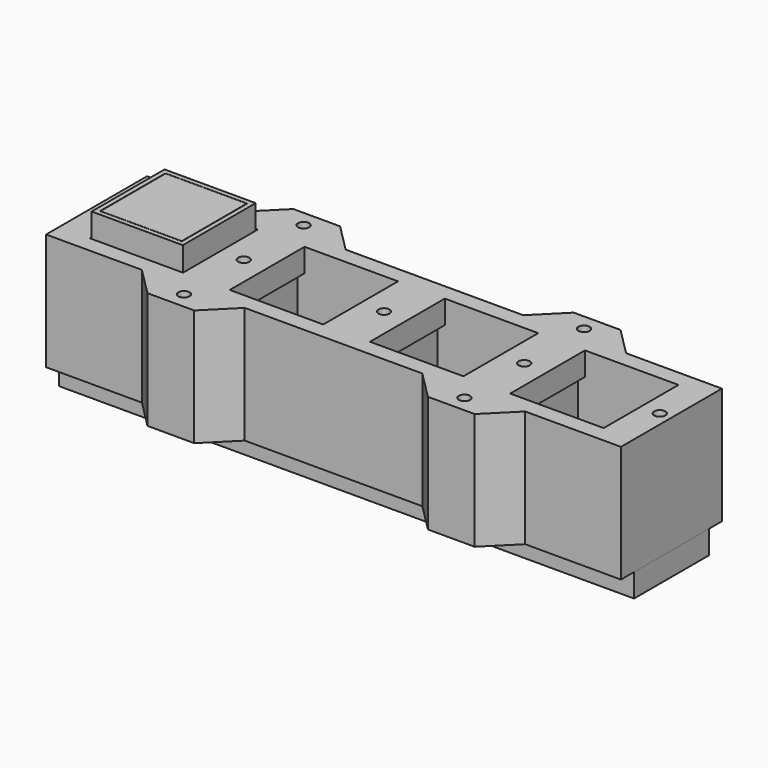
from build123d import *

# Parameters (mm, degrees)
F0_W      = 19.5
F0_H      = 19.5
F1_DEPTH  = 13
F2_W      = 19.5
F2_H      = 19.5
F2_W_2    = 17.5
F2_H_2    = 17.5
F3_DEPTH  = 6
F5_DEPTH  = 4
F6_R      = 3.1
F7_DEPTH  = 19
F8_W      = 1.5
F8_H      = 19.5
F9_DEPTH  = 9
F10_R     = 2.55
F11_DEPTH = 3
F13_W     = 10
F13_H     = 6
F13_W_2   = 20
F13_H_2   = 20
F14_DEPTH = 25
F15_W     = 23
F15_H     = 20
F16_DEPTH = 20
F17_R     = 1.2
F18_DEPTH = 30
F19_R     = 1.2
F20_DEPTH = 30.001
F21_W     = 123
F21_H     = 20
F21_R     = 2.75
F21_R_2   = 1.5
F21_R_3   = 4
F22_DEPTH = 5
F23_SIZE  = 5.99999
F25_W     = 3
F25_H     = 8
F25_H_2   = 3
F25_W_2   = 9.5
F26_DEPTH = 11
F27_W     = 17.4
F27_H     = 17.4
F28_DEPTH = 2


# Not quite as in the source:
# - a fillet or chamfer is up to 0.001 mm smaller than in the source, because OpenCascade refuses the exact size


with BuildPart() as f1:
    # F0 (on Top) → F1 (new body)
    with BuildSketch(Plane.XY):
        Rectangle(F0_W, F0_H)
    extrude(amount=F1_DEPTH)

    # F2 (on face) → F3 (join)
    with BuildSketch(Plane.XY.offset(13)):
        Rectangle(F2_W, F2_H)
        Rectangle(F2_W_2, F2_H_2, mode=Mode.SUBTRACT)
    extrude(amount=F3_DEPTH)

    # F4 (on face) → F5 (join)
    with BuildSketch(Plane.XY.offset(13)):
        Polygon((0.5, 8.75), (-0.5, 8.75), (-0.5, 0.5), (-8.75, 0.5), (-8.75, -0.5), (-0.5, -0.5), (-0.5, -8.75), (0.5, -8.75), (0.5, -0.5), (8.75, -0.5), (8.75, 0.5), (0.5, 0.5), align=None)
    extrude(amount=F5_DEPTH)

    # F6 (on face) → F7 (cut)
    with BuildSketch(Plane.XY.offset(13)):
        with Locations((-4.5, 4.5)):
            Circle(F6_R)
        with Locations((-4.5, -4.5)):
            Circle(F6_R)
        with Locations((4.5, 4.5)):
            Circle(F6_R)
        with Locations((4.5, -4.5)):
            Circle(F6_R)
    extrude(amount=-F7_DEPTH, mode=Mode.SUBTRACT)

    # F8 (on face) → F9 (join)
    with BuildSketch(Plane(origin=(0, 0, 0), x_dir=(1, 0, 0), z_dir=(0, 0, -1))):
        with Locations((-10.5, 0)):
            Rectangle(F8_W, F8_H)
        with Locations((10.5, 0)):
            Rectangle(F8_W, F8_H)
    extrude(amount=-F9_DEPTH)

    # F10 (on face) → F11 (cut)
    with BuildSketch(Plane(origin=(0, 0, 0), x_dir=(1, 0, 0), z_dir=(0, 0, -1))):
        Circle(F10_R)
    extrude(amount=-F11_DEPTH, mode=Mode.SUBTRACT)


with BuildPart() as f14:
    # F13 (on offset) → F14 (new body)
    with BuildSketch(Plane.XY.offset(14)):
        with Locations((15, 16.5)):
            Rectangle(F13_W, F13_H)
        Polygon((20, 13.5), (10, 13.5), (-16.5, 13.5), (-16.5, -13.5), (10, -13.5), (20, -13.5), (70, -13.5), (80, -13.5), (106.5, -13.5), (106.5, 13.5), (80, 13.5), (70, 13.5), align=None)
        Rectangle(F13_W_2, F13_H_2, mode=Mode.SUBTRACT)
        with Locations((30, 0)):
            Rectangle(F13_W_2, F13_H_2, mode=Mode.SUBTRACT)
        with Locations((60, 0)):
            Rectangle(F13_W_2, F13_H_2, mode=Mode.SUBTRACT)
        with Locations((90, 0)):
            Rectangle(F13_W_2, F13_H_2, mode=Mode.SUBTRACT)
        with Locations((75, 16.5)):
            Rectangle(F13_W, F13_H)
        with Locations((15, -16.5)):
            Rectangle(F13_W, F13_H)
        with Locations((75, -16.5)):
            Rectangle(F13_W, F13_H)
    extrude(amount=-F14_DEPTH)

    # F15 (on face) → F16 (cut)
    with BuildSketch(Plane(origin=(0, 0, -11), x_dir=(1, 0, 0), z_dir=(0, 0, -1))):
        Rectangle(F15_W, F15_H)
        with Locations((30, 0)):
            Rectangle(F15_W, F15_H)
        with Locations((60, 0)):
            Rectangle(F15_W, F15_H)
        with Locations((90, 0)):
            Rectangle(F15_W, F15_H)
    extrude(amount=-F16_DEPTH, mode=Mode.SUBTRACT)

    # F17 (on face) → F18 (cut)
    with BuildSketch(Plane.XY.offset(14)):
        with Locations((15, 16)):
            Circle(F17_R)
        with Locations((15, -16)):
            Circle(F17_R)
        with Locations((75, 16)):
            Circle(F17_R)
        with Locations((75, -16)):
            Circle(F17_R)
    extrude(amount=-F18_DEPTH, mode=Mode.SUBTRACT)

    # F19 (on face) → F20 (cut, through all)
    with BuildSketch(Plane(origin=(0, 0, -11), x_dir=(1, 0, 0), z_dir=(0, 0, -1))):
        with Locations((-14, 0)):
            Circle(F19_R)
        with Locations((15, 0)):
            Circle(F19_R)
        with Locations((45, 0)):
            Circle(F19_R)
        with Locations((75, 0)):
            Circle(F19_R)
        with Locations((104, 0)):
            Circle(F19_R)
    extrude(amount=-F20_DEPTH, mode=Mode.SUBTRACT)

    # F23 (size 6 in the source; OpenCascade refuses exactly that, so slightly less here)
    f23_edges = [f14.edges().sort_by_distance(p)[0] for p in [
        (10, -13.5, 1.5),
        (20, -13.5, 1.5),
        (70, -13.5, 1.5),
        (80, -13.5, 1.5),
        (10, 13.5, 1.5),
        (20, 13.5, 1.5),
        (70, 13.5, 1.5),
        (80, 13.5, 1.5),
    ]]
    chamfer(f23_edges, length=F23_SIZE)


with BuildPart() as f22:
    # F21 (on face) → F22 (new body)
    with BuildSketch(Plane(origin=(0, 0, -11), x_dir=(1, 0, 0), z_dir=(0, 0, -1))):
        with Locations((45, 0)):
            Rectangle(F21_W, F21_H)
        with Locations((-5.5, -5.5)):
            Circle(F21_R, mode=Mode.SUBTRACT)
        with Locations((5.5, -5.5)):
            Circle(F21_R, mode=Mode.SUBTRACT)
        with Locations((24.5, -5.5)):
            Circle(F21_R, mode=Mode.SUBTRACT)
        with Locations((35.5, -5.5)):
            Circle(F21_R, mode=Mode.SUBTRACT)
        with Locations((54.5, -5.5)):
            Circle(F21_R, mode=Mode.SUBTRACT)
        with Locations((65.5, -5.5)):
            Circle(F21_R, mode=Mode.SUBTRACT)
        with Locations((84.5, -5.5)):
            Circle(F21_R, mode=Mode.SUBTRACT)
        with Locations((95.5, -5.5)):
            Circle(F21_R, mode=Mode.SUBTRACT)
        with Locations((-14, 0)):
            Circle(F21_R_2, mode=Mode.SUBTRACT)
        Circle(F21_R_3, mode=Mode.SUBTRACT)
        with Locations((15, 0)):
            Circle(F21_R_2, mode=Mode.SUBTRACT)
        with Locations((30, 0)):
            Circle(F21_R_3, mode=Mode.SUBTRACT)
        with Locations((-5.5, 5.5)):
            Circle(F21_R, mode=Mode.SUBTRACT)
        with Locations((5.5, 5.5)):
            Circle(F21_R, mode=Mode.SUBTRACT)
        with Locations((24.5, 5.5)):
            Circle(F21_R, mode=Mode.SUBTRACT)
        with Locations((35.5, 5.5)):
            Circle(F21_R, mode=Mode.SUBTRACT)
        with Locations((45, 0)):
            Circle(F21_R_2, mode=Mode.SUBTRACT)
        with Locations((60, 0)):
            Circle(F21_R_3, mode=Mode.SUBTRACT)
        with Locations((75, 0)):
            Circle(F21_R_2, mode=Mode.SUBTRACT)
        with Locations((90, 0)):
            Circle(F21_R_3, mode=Mode.SUBTRACT)
        with Locations((104, 0)):
            Circle(F21_R_2, mode=Mode.SUBTRACT)
        with Locations((54.5, 5.5)):
            Circle(F21_R, mode=Mode.SUBTRACT)
        with Locations((65.5, 5.5)):
            Circle(F21_R, mode=Mode.SUBTRACT)
        with Locations((84.5, 5.5)):
            Circle(F21_R, mode=Mode.SUBTRACT)
        with Locations((95.5, 5.5)):
            Circle(F21_R, mode=Mode.SUBTRACT)
    extrude(amount=F22_DEPTH)


with BuildPart() as f26:
    # F25 (on offset) → F26 (new body)
    with BuildSketch(Plane(origin=(0, 0, -11), x_dir=(1, 0, 0), z_dir=(0, 0, -1))):
        with Locations((0, -5.5)):
            Rectangle(F25_W, F25_H)
        Rectangle(F25_W, F25_H_2)
        with Locations((6.25, 0)):
            Rectangle(F25_W_2, F25_H_2)
        with Locations((-6.25, 0)):
            Rectangle(F25_W_2, F25_H_2)
        with Locations((0, 5.5)):
            Rectangle(F25_W, F25_H)
    extrude(amount=-F26_DEPTH)


with BuildPart() as f28:
    # F27 (on face) → F28 (new body)
    with BuildSketch(Plane.XY.offset(19)):
        Rectangle(F27_W, F27_H)
    extrude(amount=-F28_DEPTH)


solid = Compound([f1.part, f14.part, f22.part, f26.part, f28.part])
